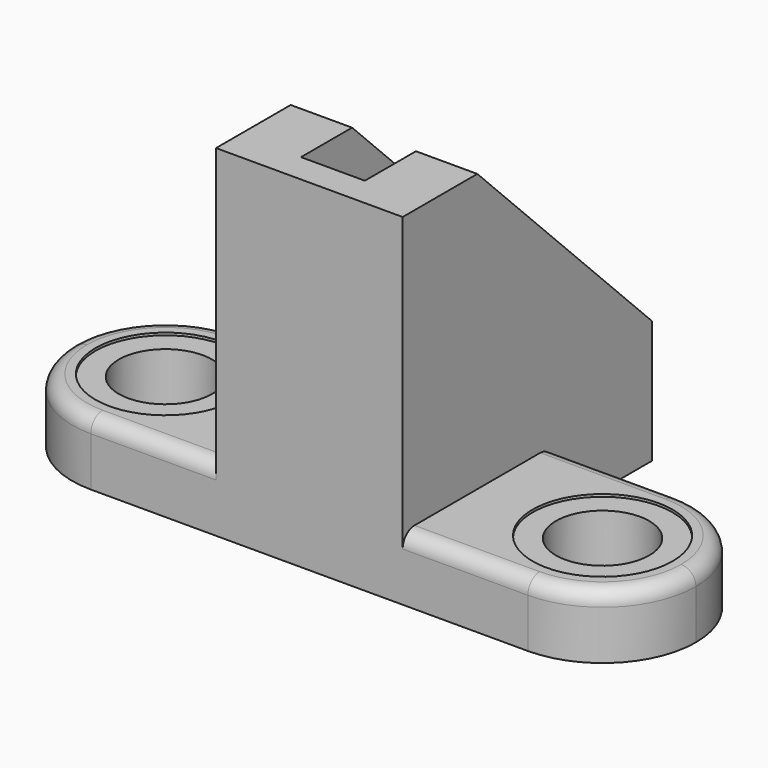
from build123d import *

# Parameters (mm, degrees)
F1_DEPTH  = 25
F3_DEPTH  = 13
F4_W      = 76
F4_H      = 26
F5_DEPTH  = 89
F7_DEPTH  = 26.001
F9_R      = 19
F10_DEPTH = 26.001
F9_R_2    = 28.5
F11_DEPTH = 1
F12_R     = 6


with BuildPart() as f1:
    # F0 (on Right) → F1 (new body)
    with BuildSketch(Plane.YZ):
        Polygon((-127, 0), (0, 0), (0, 50), (-89, 139), (-127, 139), align=None)
    extrude(amount=F1_DEPTH)

    # F2 (on face) → F3 (join)
    with BuildSketch(Plane(origin=(0, 0, 0), x_dir=(0, -1, 0), z_dir=(-1, 0, 0))):
        Polygon((0, 24), (0, 0), (127, 0), (127, 139), (115, 139), align=None)
    extrude(amount=F3_DEPTH)

    # F4 (on face) → F5 (join)
    with BuildSketch(Plane.YZ.offset(25)):
        with Locations((-89, 13)):
            Rectangle(F4_W, F4_H)
    extrude(amount=F5_DEPTH)

    # F6 (on face) → F7 (cut, through all)
    with BuildSketch(Plane.XY.offset(26)):
        with BuildLine():
            ThreePointArc((76, -51), (102.8700576851, -62.1299423149), (114, -89))
            Line((114, -89), (114, -51))
            Line((114, -51), (76, -51))
        make_face()
        with BuildLine():
            Line((114, -127), (114, -89))
            ThreePointArc((114, -89), (102.8700576851, -115.8700576851), (76, -127))
            Line((76, -127), (114, -127))
        make_face()
    extrude(amount=-F7_DEPTH, mode=Mode.SUBTRACT)

    # F9 (on face) → F10 (cut, through all)
    with BuildSketch(Plane.XY.offset(26)):
        with Locations((76, -89)):
            Circle(F9_R)
    extrude(amount=-F10_DEPTH, mode=Mode.SUBTRACT)

    # F9 (on face) → F11 (cut)
    with BuildSketch(Plane.XY.offset(26)):
        with Locations((76, -89)):
            Circle(F9_R_2)
        with Locations((76, -89)):
            Circle(F9_R, mode=Mode.SUBTRACT)
    extrude(amount=-F11_DEPTH, mode=Mode.SUBTRACT)

    # F12
    f12_edges = [f1.edges().sort_by_distance(p)[0] for p in [
        (50.5, -51, 26),
        (50.5, -127, 26),
        (114, -89, 26),
    ]]
    fillet(f12_edges, radius=F12_R)

    # F13: F1 across plane


with BuildPart() as f1_1:
    add(f1.part)
    add(f1.part.mirror(Plane.YZ.offset(-13)))


solid = f1_1.part
